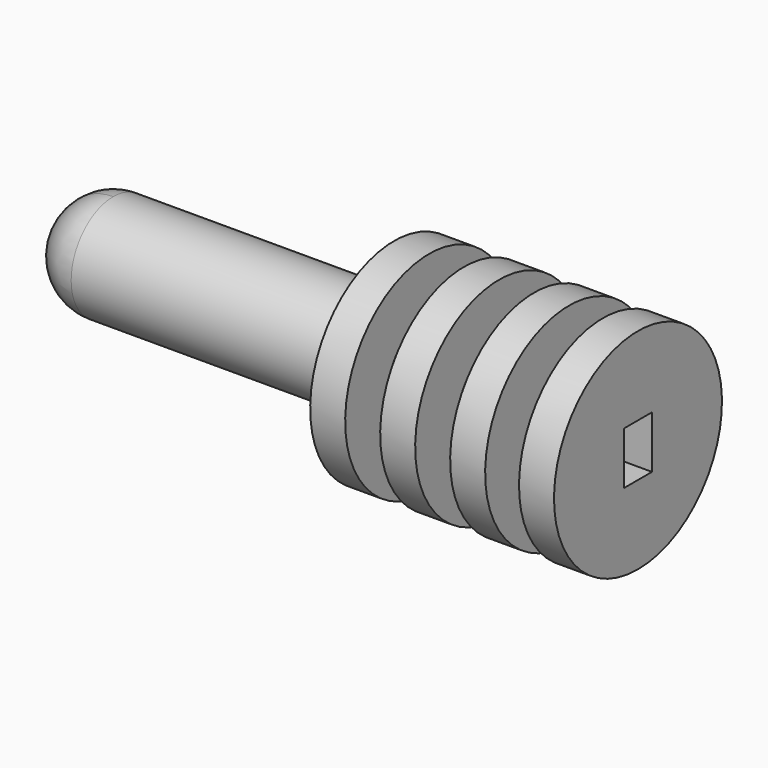
from build123d import *
from build123d import SkipClean  # not in build123d's __all__

# Parameters (mm, degrees)
F1_W     = 10
F1_H     = 15
F3_W     = 10
F3_H     = 15
F5_DEPTH = 15


with BuildPart() as f2:
    # F1 (on Front) → F2 (revolve)
    with BuildSketch(Plane.XZ):
        Polygon((150, -15), (150, 0), (140.3131330013, 0), (140, -15), align=None)
        Polygon((138.0902081728, 15), (0, 15), (0, 0), (80.3131330013, 0), (90.3131330013, 0), (100.3131330013, 0), (110.3131330013, 0), (120.3131330013, 0), (130.3131330013, 0), (140.3131330013, 0), (150, 0), (150, 15), align=None)
        with Locations((125.3131330013, -7.5)):
            Rectangle(F1_W, F1_H)
        with Locations((105.3131330013, -7.5)):
            Rectangle(F1_W, F1_H)
        with Locations((85.3131330013, -7.5)):
            Rectangle(F1_W, F1_H)
    revolve(axis=Axis((75, 0, 15), (1, 0, 0)))

    # F0 (on Front) → F4 (revolve)
    with BuildSketch(Plane.XZ):
        with BuildLine():
            ThreePointArc((0, 30), (-15, 15), (0, 0))
            Line((0, 0), (0, 30))
        make_face()
    with SkipClean():  # cleaning this boolean's faces spoils the solid; the shape is the same uncleaned
        revolve(axis=Axis((0, 0, 15), (0, 0, 1)))

    # F3 (on face) → F5 (cut)
    with BuildSketch(Plane.YZ.offset(150)):
        with Locations((0, 15)):
            Rectangle(F3_W, F3_H)
    with SkipClean():  # cleaning this boolean's faces spoils the solid; the shape is the same uncleaned
        extrude(amount=-F5_DEPTH, mode=Mode.SUBTRACT)


solid = f2.part
